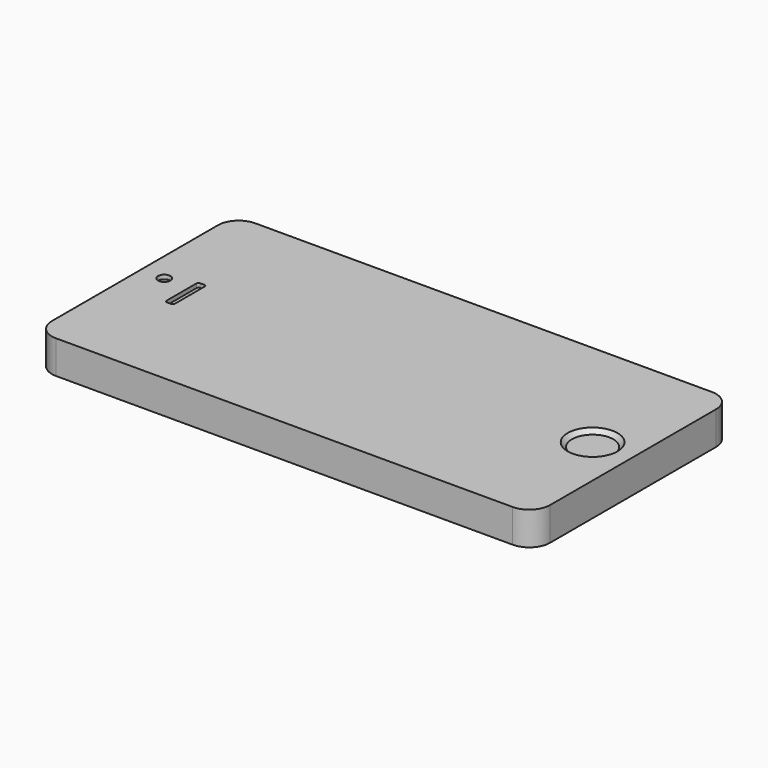
from build123d import *

# Parameters (mm, degrees)
F0_W      = 120
F0_H      = 60
F1_DEPTH  = 8
F2_R      = 5
F3_R      = 5
F4_R      = 5
F5_R      = 5
F6_W      = 2
F6_H      = 10
F7_DEPTH  = 1
F8_R      = 0.5
F9_R      = 0.5
F10_R     = 1.5
F11_DEPTH = 1
F14_R     = 6
F15_DEPTH = 1
F16_SIZE  = 0.99999


# Not quite as in the source:
# - a fillet or chamfer is up to 0.001 mm smaller than in the source, because OpenCascade refuses the exact size


with BuildPart() as f1:
    # F0 (on Top) → F1 (new body)
    with BuildSketch(Plane.XY):
        with Locations((60, 30)):
            Rectangle(F0_W, F0_H)
    extrude(amount=F1_DEPTH)

    # F2
    f2_edges = [f1.edges().sort_by_distance(p)[0] for p in [
        (0, 60, 4),
    ]]
    fillet(f2_edges, radius=F2_R)

    # F3
    f3_edges = [f1.edges().sort_by_distance(p)[0] for p in [
        (0, 0, 4),
    ]]
    fillet(f3_edges, radius=F3_R)

    # F4
    f4_edges = [f1.edges().sort_by_distance(p)[0] for p in [
        (120, 0, 4),
    ]]
    fillet(f4_edges, radius=F4_R)

    # F5
    f5_edges = [f1.edges().sort_by_distance(p)[0] for p in [
        (120, 60, 4),
    ]]
    fillet(f5_edges, radius=F5_R)

    # F6 (on face) → F7 (cut)
    with BuildSketch(Plane.XY.offset(8)):
        with Locations((12.6586212461, 29.4524356723)):
            Rectangle(F6_W, F6_H)
    extrude(amount=-F7_DEPTH, mode=Mode.SUBTRACT)

    # F8
    f8_edges = [f1.edges().sort_by_distance(p)[0] for p in [
        (11.658621, 24.452436, 7.5),
        (13.658621, 24.452436, 7.5),
    ]]
    fillet(f8_edges, radius=F8_R)

    # F9
    f9_edges = [f1.edges().sort_by_distance(p)[0] for p in [
        (13.658621, 34.452436, 7.5),
        (11.658621, 34.452436, 7.5),
    ]]
    fillet(f9_edges, radius=F9_R)

    # F10 (on face) → F11 (cut)
    with BuildSketch(Plane.XY.offset(8)):
        with Locations((5.6273336522, 31.8058170378)):
            Circle(F10_R)
    extrude(amount=-F11_DEPTH, mode=Mode.SUBTRACT)

    # F14 (on face) → F15 (cut)
    with BuildSketch(Plane.XY.offset(8)):
        with Locations((110.2445796132, 30)):
            Circle(F14_R)
    extrude(amount=-F15_DEPTH, mode=Mode.SUBTRACT)

    # F16 (size 1 in the source; OpenCascade refuses exactly that, so slightly less here)
    f16_edges = [f1.edges().sort_by_distance(p)[0] for p in [
        (104.24458, 30, 7),
    ]]
    chamfer(f16_edges, length=F16_SIZE)


solid = f1.part
